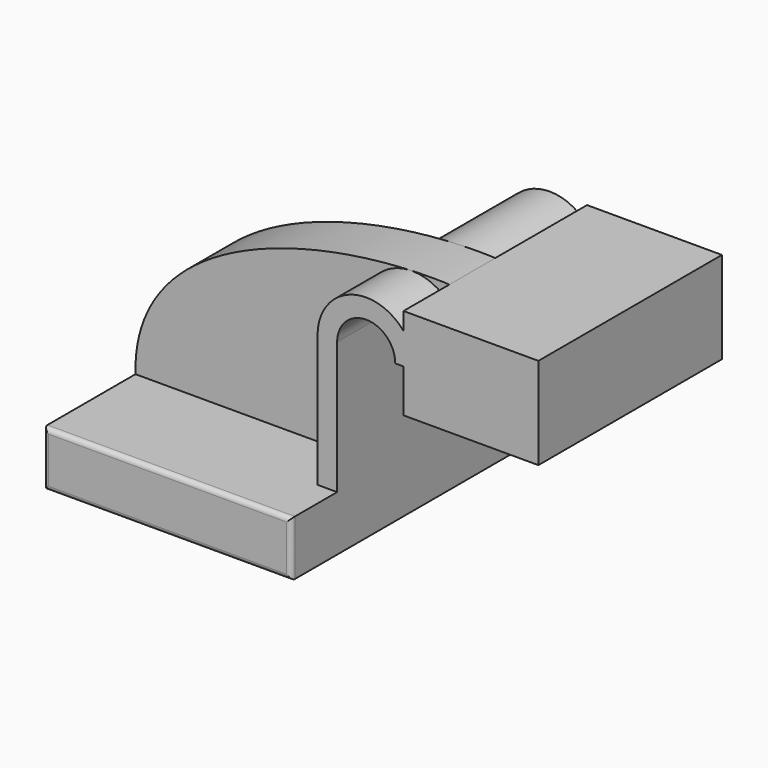
from build123d import *

# Parameters (mm, degrees)
F2_DEPTH = 50
F3_DEPTH = 25
F4_DEPTH = 25
F6_DEPTH = 75
F7_R     = 2


# Not quite as in the source:
# - the program builds the solid bodies; features that only make, move or delete a surface that nothing else refers to are left out


with BuildPart() as f2:
    # F0 (on Front) → F2 (new body, symmetric)
    with BuildSketch(Plane.XZ):
        with BuildLine():
            ThreePointArc((86.0395411487, 78.1614595205), (84.6450154703, 80.8109382584), (82.8911252312, 83.2375219638))
            Line((82.8911252312, 83.2375219638), (82.8911252312, 69.6372875124))
            Line((82.8911252312, 69.6372875124), (98.3350202441, 69.6372875124))
            Line((98.3350202441, 69.6372875124), (98.3350202441, 78.1614595205))
            Line((98.3350202441, 78.1614595205), (86.0395411487, 78.1614595205))
        make_face()
        with BuildLine():
            Line((141.6950114063, 90.9081755561), (82.8911252312, 90.9081755561))
            Line((82.8911252312, 90.9081755561), (82.8911252312, 83.2375219638))
            ThreePointArc((82.8911252312, 83.2375219638), (84.6450154703, 80.8109382584), (86.0395411487, 78.1614595205))
            Line((86.0395411487, 78.1614595205), (98.3350202441, 78.1614595205))
            Line((98.3350202441, 78.1614595205), (98.3350202441, 69.6372875124))
            Line((98.3350202441, 69.6372875124), (82.8911252312, 69.6372875124))
            Line((82.8911252312, 69.6372875124), (82.8911252312, 50.8714897913))
            Line((82.8911252312, 50.8714897913), (141.6950114063, 50.8714897913))
            Line((141.6950114063, 50.8714897913), (141.6950114063, 90.9081755561))
        make_face()
        with BuildLine():
            Line((45.431509614, 69.6372875124), (45.431509614, 12))
            Line((45.431509614, 12), (53.955681622, 12))
            Line((53.955681622, 12), (53.955681622, 69.6372875124))
            ThreePointArc((53.955681622, 69.6372875124), (66.6301945598, 82.3118004502), (79.3047074976, 69.6372875124))
            Line((79.3047074976, 69.6372875124), (82.8911252312, 69.6372875124))
            Line((82.8911252312, 69.6372875124), (82.8911252312, 83.2375219638))
            ThreePointArc((82.8911252312, 83.2375219638), (59.3957665519, 89.563333152), (45.431509614, 69.6372875124))
        make_face()
    extrude(amount=F2_DEPTH, both=True)

    # F0 (on Front) → F3 (join)
    with BuildSketch(Plane.XZ):
        with BuildLine():
            add(Edge.make_bspline(
                [(-53.955681622, 12), (-55.4214757867, 72.6385811269), (29.6854469925, 93.0915244818), (82.8911252312, 90.9081755561)],
                knots=[0, 0, 0, 0, 157.9669228526, 157.9669228526, 157.9669228526, 157.9669228526], degree=3))
            Line((-53.955681622, 12), (45.431509614, 12))
            Line((45.431509614, 12), (45.431509614, 69.6372875124))
            ThreePointArc((45.431509614, 69.6372875124), (59.3957665519, 89.563333152), (82.8911252312, 83.2375219638))
            Line((82.8911252312, 83.2375219638), (82.8911252312, 90.9081755561))
        make_face()
        Polygon((45.431509614, 12), (-53.955681622, 12), (-53.955681622, -12), (53.955681622, -12), (53.955681622, 12), align=None)
        with BuildLine():
            Line((45.431509614, 69.6372875124), (45.431509614, 12))
            Line((45.431509614, 12), (53.955681622, 12))
            Line((53.955681622, 12), (53.955681622, 69.6372875124))
            ThreePointArc((53.955681622, 69.6372875124), (66.6301945598, 82.3118004502), (79.3047074976, 69.6372875124))
            Line((79.3047074976, 69.6372875124), (82.8911252312, 69.6372875124))
            Line((82.8911252312, 69.6372875124), (82.8911252312, 83.2375219638))
            ThreePointArc((82.8911252312, 83.2375219638), (59.3957665519, 89.563333152), (45.431509614, 69.6372875124))
        make_face()
        with BuildLine():
            Line((141.6950114063, 90.9081755561), (82.8911252312, 90.9081755561))
            Line((82.8911252312, 90.9081755561), (82.8911252312, 83.2375219638))
            ThreePointArc((82.8911252312, 83.2375219638), (84.6450154703, 80.8109382584), (86.0395411487, 78.1614595205))
            Line((86.0395411487, 78.1614595205), (98.3350202441, 78.1614595205))
            Line((98.3350202441, 78.1614595205), (98.3350202441, 69.6372875124))
            Line((98.3350202441, 69.6372875124), (82.8911252312, 69.6372875124))
            Line((82.8911252312, 69.6372875124), (82.8911252312, 50.8714897913))
            Line((82.8911252312, 50.8714897913), (141.6950114063, 50.8714897913))
            Line((141.6950114063, 50.8714897913), (141.6950114063, 90.9081755561))
        make_face()
        with BuildLine():
            ThreePointArc((86.0395411487, 78.1614595205), (84.6450154703, 80.8109382584), (82.8911252312, 83.2375219638))
            Line((82.8911252312, 83.2375219638), (82.8911252312, 69.6372875124))
            Line((82.8911252312, 69.6372875124), (98.3350202441, 69.6372875124))
            Line((98.3350202441, 69.6372875124), (98.3350202441, 78.1614595205))
            Line((98.3350202441, 78.1614595205), (86.0395411487, 78.1614595205))
        make_face()
    extrude(amount=F3_DEPTH)

    # F0 (on Front) → F4 (join, symmetric)
    with BuildSketch(Plane.XZ):
        Polygon((45.431509614, 12), (-53.955681622, 12), (-53.955681622, -12), (53.955681622, -12), (53.955681622, 12), align=None)
    extrude(amount=F4_DEPTH, both=True)

    # F1 (on face) → F6 (join, symmetric)
    with BuildSketch(Plane.XZ):
        Polygon((53.955681622, 12), (45.431509614, 12), (-53.955681622, 12), (-53.955681622, -12), (53.955681622, -12), align=None)
    extrude(amount=F6_DEPTH, both=True)

    # F7
    f7_edges = [f2.edges().sort_by_distance(p)[0] for p in [
        (53.955682, -75, 0),
        (0, -75, 12),
        (-53.955682, -75, 0),
        (0, -75, -12),
        (53.955682, 75, 0),
        (0, 75, 12),
        (-53.955682, 75, 0),
        (0, 75, -12),
    ]]
    fillet(f7_edges, radius=F7_R)


solid = f2.part
